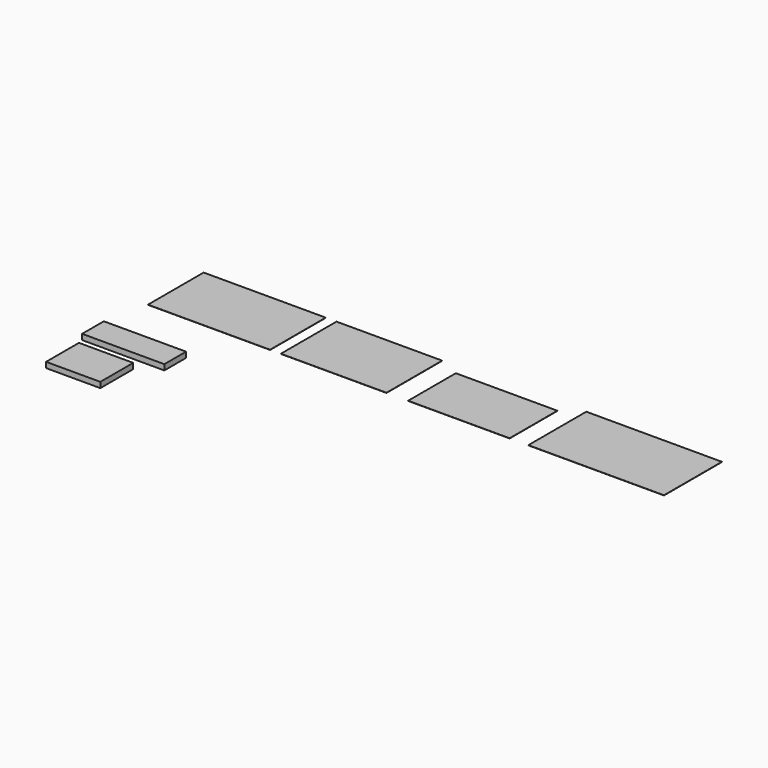
from build123d import *

# Parameters (mm, degrees)
F0_W     = 2970
F0_H     = 1692
F1_DEPTH = 5
F0_W_2   = 2570
F0_W_3   = 2470
F0_H_2   = 1450
F0_W_4   = 3300
F0_H_3   = 1762
F0_W_5   = 2000
F0_H_4   = 660
F2_DEPTH = 135
F0_W_6   = 1320
F0_H_5   = 1000


with BuildPart() as f1:
    # F0 (on Top) → F1 (new body)
    with BuildSketch(Plane.XY):
        with Locations((1416.5291196108, 896.7160201669)):
            Rectangle(F0_W, F0_H)
    extrude(amount=F1_DEPTH)


with BuildPart() as f1b:
    # F0 (on Top) → F1, piece 2 (new body)
    with BuildSketch(Plane.XY):
        with Locations((4449.041519165, 896.7160201669)):
            Rectangle(F0_W_2, F0_H)
    extrude(amount=F1_DEPTH)


with BuildPart() as f1c:
    # F0 (on Top) → F1, piece 3 (new body)
    with BuildSketch(Plane.XY):
        with Locations((7495.8523368835, 775.7160201669)):
            Rectangle(F0_W_3, F0_H_2)
    extrude(amount=F1_DEPTH)


with BuildPart() as f1d:
    # F0 (on Top) → F1, piece 4 (new body)
    with BuildSketch(Plane.XY):
        with Locations((10835.6288909912, 931.7160201669)):
            Rectangle(F0_W_4, F0_H_3)
    extrude(amount=F1_DEPTH)


with BuildPart() as f2:
    # F0 (on Top) → F2 (new body)
    with BuildSketch(Plane.XY):
        with Locations((860.1830005646, -1533.1247282028)):
            Rectangle(F0_W_5, F0_H_4)
    extrude(amount=F2_DEPTH)


with BuildPart() as f2b:
    # F0 (on Top) → F2, piece 2 (new body)
    with BuildSketch(Plane.XY):
        with Locations((705.0170564651, -2691.0228729248)):
            Rectangle(F0_W_6, F0_H_5)
    extrude(amount=F2_DEPTH)


solid = Compound([f1.part, f1b.part, f1c.part, f1d.part, f2.part, f2b.part])
